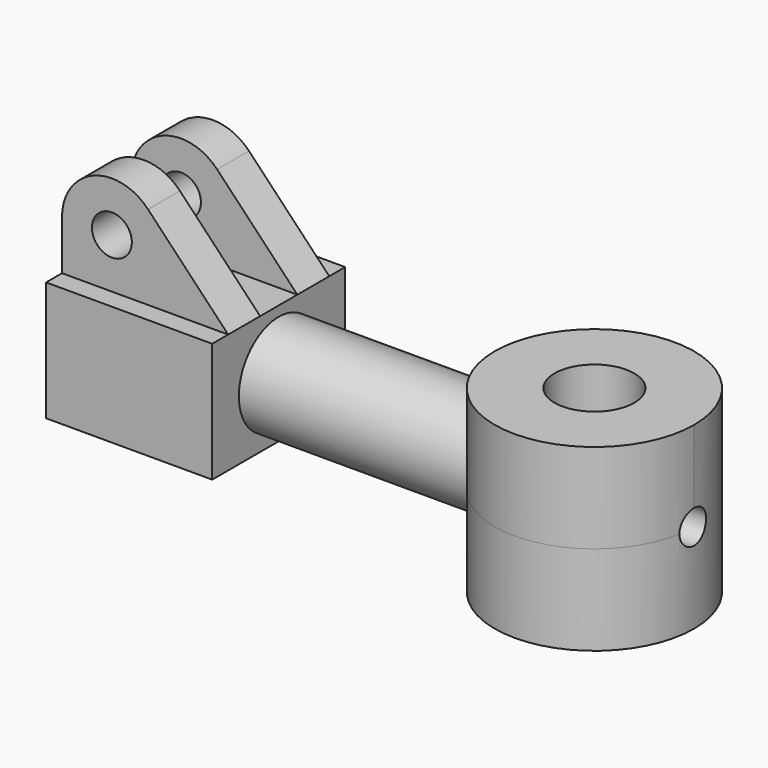
from build123d import *

# Parameters (mm, degrees)
F0_R     = 6
F1_DEPTH = 18
F0_R_2   = 12
F3_DEPTH = 27
F4_R     = 5
F5_DEPTH = 175.0010001
F7_R     = 6
F8_DEPTH = 12


# Not quite as in the source:
# - a pattern or mirror of a feature is missing from the dataset's text; its kind, count and spacing are read off the source's solid


with BuildPart() as f1:
    # F0 (on Top) → F1 (new body, symmetric)
    with BuildSketch(Plane.XY):
        Polygon((25, 15), (25, 25), (-25, 25), (-25, -25), (25, -25), (25, 0), align=None)
        Circle(F0_R, mode=Mode.SUBTRACT)
    extrude(amount=F1_DEPTH, both=True)

    # F0 (on Top) → F2 (revolve)
    with BuildSketch(Plane.XY):
        with BuildLine():
            Line((94.0192378865, 15), (25, 15))
            Line((25, 15), (25, 0))
            Line((25, 0), (90, 0))
            ThreePointArc((90, 0), (91.0222252113, 7.7645713531), (94.0192378865, 15))
        make_face()
    revolve(axis=Axis((57.5, 0, 0), (1, 0, 0)))

    # F0 (on Top) → F3 (join, symmetric)
    with BuildSketch(Plane.XY):
        with BuildLine():
            ThreePointArc((150, 0), (127.7645713531, 28.9777747887), (94.0192378865, 15))
            ThreePointArc((94.0192378865, 15), (91.0222252113, 7.7645713531), (90, 0))
            ThreePointArc((90, 0), (120, -30), (150, 0))
        make_face()
        with Locations((120, 0)):
            Circle(F0_R_2, mode=Mode.SUBTRACT)
    extrude(amount=F3_DEPTH, both=True)

    # F4 (on face) → F5 (cut, through all)
    with BuildSketch(Plane(origin=(-25, 0, 0), x_dir=(0, -1, 0), z_dir=(-1, 0, 0))):
        Circle(F4_R)
    extrude(amount=-F5_DEPTH, mode=Mode.SUBTRACT)

    # F7 (on offset) → F8 (join)
    with BuildSketch(Plane(origin=(0, 19, 0), x_dir=(-1, 0, 0), z_dir=(0, 1, 0))):
        with BuildLine():
            Line((25, 18), (25, 33))
            ThreePointArc((25, 33), (15.5708601453, 46.9271503633), (-0.8620689655, 43.3448275862))
            Line((-0.8620689655, 43.3448275862), (-25, 18))
            Line((-25, 18), (25, 18))
        make_face()
        with Locations((10, 33)):
            Circle(F7_R, mode=Mode.SUBTRACT)
    f8 = extrude(amount=-F8_DEPTH)

    # F8_copies: F8 across plane
    add(f8.mirror(Plane(origin=(0, 0, 0), x_dir=(0, 0, -1), z_dir=(0, -1, 0))))


solid = f1.part
